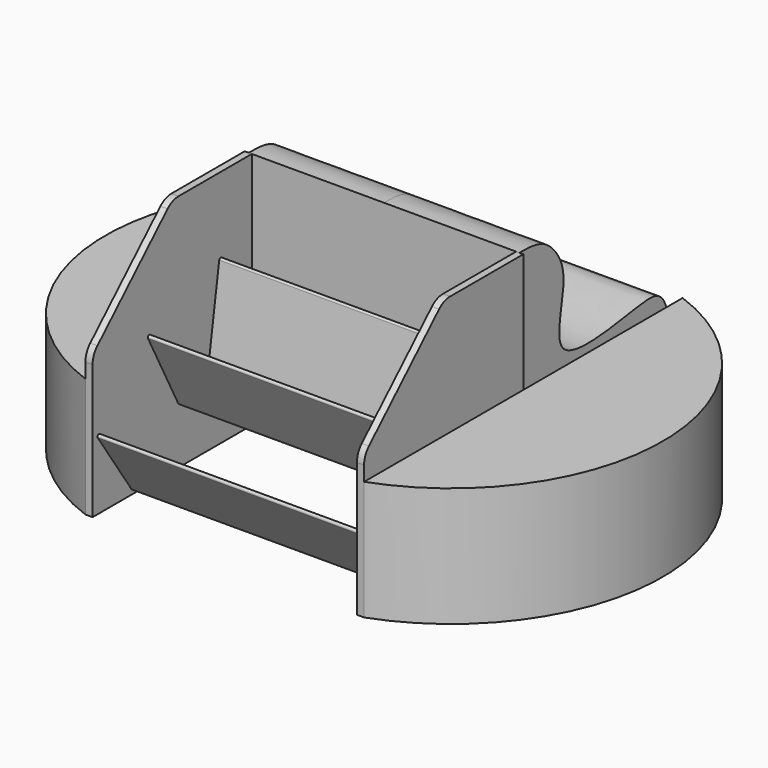
from build123d import *

# Parameters (mm, degrees)
F1_DEPTH      = 30
F3_DEPTH      = 34
F3_DEPTH_BACK = 34
F5_DEPTH      = 1.8
F8_DEPTH      = 66.4


with BuildPart() as f1:
    # F0 (on Top) → F1 (new body)
    with BuildSketch(Plane.XY):
        with BuildLine():
            Line((-35, -50), (-35, 50))
            ThreePointArc((-35, 50), (-70, 0), (-35, -50))
        make_face()
    extrude(amount=F1_DEPTH)


with BuildPart() as f1b:
    # F0 (on Top) → F1, piece 2 (new body)
    with BuildSketch(Plane.XY):
        with BuildLine():
            ThreePointArc((35, -50), (70, 0), (35, 50))
            Line((35, 50), (35, -50))
        make_face()
    extrude(amount=F1_DEPTH)


with BuildPart() as f3:
    # F2 (on Right) → F3 (new body, two sides)
    with BuildSketch(Plane.YZ) as f3_sk:
        with BuildLine():
            Line((0, 60), (0, 0))
            Line((0, 0), (49.5640300214, 0))
            add(Edge.make_bspline(
                [(0, 60), (6.0089451636, 60.144637794), (10.3960435461, 57.7340089425), (16.0813784265, 48.6153030742), (7.373119025, 27.6080491003), (37.1506971717, 33.3219817547), (46.5801176583, 33.7548207857), (48.7225614629, 14.7430900128), (49.3265567032, 4.8876965388), (49.5640300214, 0)],
                knots=[0, 0, 0, 0, 0.1271378904, 0.2453891259, 0.3945005936, 0.5798905169, 0.6907038362, 0.8468495544, 1, 1, 1, 1], degree=3))
        make_face()
    extrude(amount=F3_DEPTH)
    extrude(f3_sk.sketch, amount=-F3_DEPTH_BACK)


with BuildPart() as f5:
    # F4 (on face) → F5 (new body)
    with BuildSketch(Plane.YZ.offset(-35)):
        with BuildLine():
            Line((-50, 0), (0, 0))
            Line((0, 0), (0, 60))
            Line((0, 60), (-22.977684609, 60))
            ThreePointArc((-22.977684609, 60), (-24.8524581938, 59.6352156374), (-26.4536765438, 58.5940896022))
            Line((-26.4536765438, 58.5940896022), (-48.4759919348, 37.2954022692))
            ThreePointArc((-48.4759919348, 37.2954022692), (-49.6032575245, 35.6532399614), (-50, 33.7013126669))
            Line((-50, 33.7013126669), (-50, 0))
        make_face()
    extrude(amount=F5_DEPTH)


with BuildPart() as f6_1:
    # F6: instance of F5
    add(f5.part.mirror(Plane.YZ))


with BuildPart() as f5_1:
    add(f5.part)

    add(f6_1.part)  # F8 merges F6_1
    # F7 (on face) → F8 (join, through all)
    with BuildSketch(Plane.YZ.offset(-33.2)):
        with BuildLine():
            ThreePointArc((-31.8018199972, 32.8599235604), (-32.4088281582, 33.0510808059), (-32.5999854037, 32.4440726449))
            Line((-32.5999854037, 32.4440726449), (-23.0850910672, 14.1816155424))
            ThreePointArc((-23.0850910672, 14.1816155424), (-22.4780829062, 13.9904582969), (-22.2869256607, 14.5974664579))
            Line((-22.2869256607, 14.5974664579), (-31.8018199972, 32.8599235604))
        make_face()
        with BuildLine():
            ThreePointArc((-47.6351742196, 17.40406865), (-48.2600409698, 17.5246569764), (-48.3806292963, 16.8997902262))
            Line((-48.3806292963, 16.8997902262), (-37.7914729965, 1.2462545025))
            ThreePointArc((-37.7914729965, 1.2462545025), (-37.1666062462, 1.1256661761), (-37.0460179198, 1.7505329263))
            Line((-37.0460179198, 1.7505329263), (-47.6351742196, 17.40406865))
        make_face()
        with BuildLine():
            ThreePointArc((-9.3500294415, 40.5642331237), (-9.7268621096, 41.0770655917), (-10.2396945776, 40.7002329236))
            Line((-10.2396945776, 40.7002329236), (-13.9228713829, 16.6061240042))
            ThreePointArc((-13.9228713829, 16.6061240042), (-13.5460387148, 16.0932915362), (-13.0332062468, 16.4701242042))
            Line((-13.0332062468, 16.4701242042), (-9.3500294415, 40.5642331237))
        make_face()
    extrude(amount=F8_DEPTH)


solid = Compound([f1.part, f1b.part, f3.part, f5_1.part])
